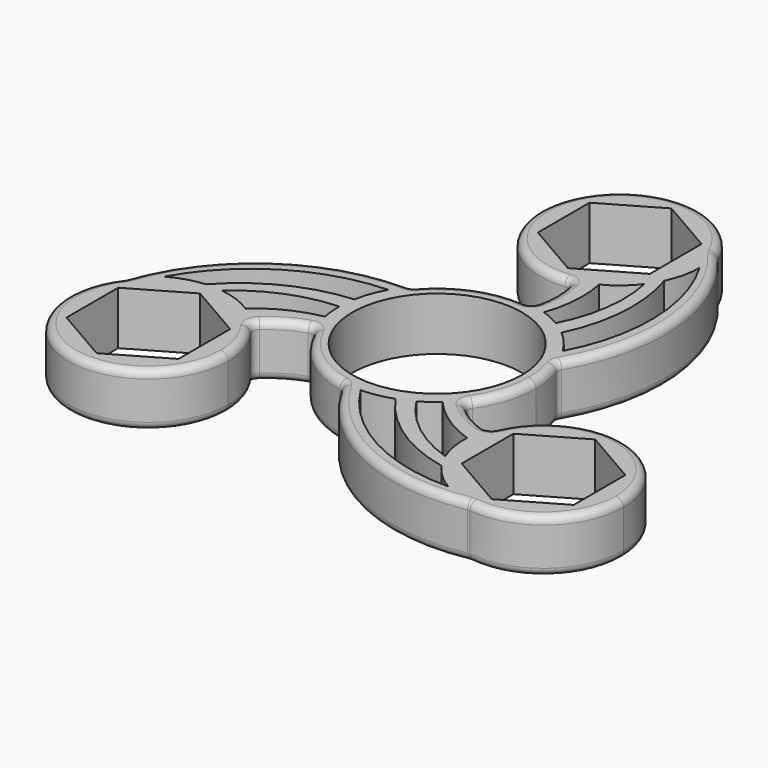
from build123d import *

# Parameters (mm, degrees)
F0_R     = 11.15
F1_DEPTH = 7
F2_R     = 1


with BuildPart() as f1:
    # F0 (on Top) → F1 (new body)
    with BuildSketch(Plane.XY):
        with BuildLine():
            ThreePointArc((-11.4217360903, 6.2083769767), (-10.7651051073, 7.2878331504), (-10.0067859301, 8.2984477674))
            ThreePointArc((-10.0067859301, 8.2984477674), (-24.8747570985, 3.8510516113), (-34.2433879176, -8.5208785455))
            ThreePointArc((-34.2433879176, -8.5208785455), (-32.8623464459, -7.069439044), (-31.2307621135, -5.9067332603))
            ThreePointArc((-31.2307621135, -5.9067332603), (-22.9201483535, 2.7569551195), (-11.4217360903, 6.2083769767))
        make_face()
        with BuildLine():
            ThreePointArc((-12.9988117388, 0.1757651253), (-12.936896451, 1.2793397577), (-12.7814596137, 2.3736659713))
            ThreePointArc((-12.7814596137, 2.3736659713), (-20.4515190805, 0.2762194234), (-26.7856148565, -4.5308924897))
            ThreePointArc((-26.7856148565, -4.5308924897), (-25.7070937202, -4.5035670054), (-24.6314618134, -4.5870566745))
            ThreePointArc((-24.6314618134, -4.5870566745), (-19.2285330831, -1.1959723533), (-12.9988117388, 0.1757651253))
        make_face()
        with BuildLine():
            ThreePointArc((-18.0539765779, -8.1140671604), (-15.3384929239, -5.9704194589), (-12.1242977306, -4.6905654818))
            ThreePointArc((-12.1242977306, -4.6905654818), (-12.4885737373, -3.6104744852), (-12.7568359951, -2.5026256999))
            ThreePointArc((-12.7568359951, -2.5026256999), (-16.7613572368, -3.8405452144), (-20.2703349988, -6.1885856886))
            ThreePointArc((-20.2703349988, -6.1885856886), (-19.0945249739, -7.0734788174), (-18.0539765779, -8.1140671604))
        make_face()
        with BuildLine():
            ThreePointArc((-31.2307621135, -5.9067332603), (-32.8623464459, -7.069439044), (-34.2433879176, -8.5208785455))
            ThreePointArc((-34.2433879176, -8.5208785455), (-29.4080372015, -24.9249073281), (-15.4807621135, -15))
            ThreePointArc((-15.4807621135, -15), (-16.1450809443, -11.3244897038), (-18.0539765779, -8.1140671604))
            ThreePointArc((-18.0539765779, -8.1140671604), (-19.0945249739, -7.0734788174), (-20.2703349988, -6.1885856886))
            ThreePointArc((-20.2703349988, -6.1885856886), (-22.3612094355, -5.143588969), (-24.6314618134, -4.5870566745))
            ThreePointArc((-24.6314618134, -4.5870566745), (-25.7070937202, -4.5035670054), (-26.7856148565, -4.5308924897))
            ThreePointArc((-26.7856148565, -4.5308924897), (-29.0853627145, -4.9694738369), (-31.2307621135, -5.9067332603))
        make_face()
        Polygon((-25.9807621135, -23.5), (-33.3419780457, -19.25), (-33.3419780457, -10.75), (-25.9807621135, -6.5), (-18.6195461814, -10.75), (-18.6195461814, -19.25), align=None, mode=Mode.SUBTRACT)
        with BuildLine():
            ThreePointArc((10.1242977306, -8.1546670969), (12.2600136725, -4.3234320569), (13, 0))
            ThreePointArc((13, 0), (12.7959129035, 2.2944744423), (12.1900595436, 4.516906942))
            ThreePointArc((12.1900595436, 4.516906942), (11.6940012005, 5.6789379222), (11.0874802232, 6.7873251211))
            ThreePointArc((11.0874802232, 6.7873251211), (9.8887607408, 8.4387446348), (8.4463848381, 9.8822357373))
            ThreePointArc((8.4463848381, 9.8822357373), (7.5763889557, 10.5640110939), (6.651622933, 11.1694186222))
            ThreePointArc((6.651622933, 11.1694186222), (5.460641215, 11.7975165828), (4.2110805653, 12.2990568936))
            ThreePointArc((4.2110805653, 12.2990568936), (3.1175242448, 12.6206593561), (2, 12.8452325787))
            ThreePointArc((2, 12.8452325787), (-4.6038536318, 12.1574887101), (-10.0067859301, 8.2984477674))
            ThreePointArc((-10.0067859301, 8.2984477674), (-10.7651051073, 7.2878331504), (-11.4217360903, 6.2083769767))
            ThreePointArc((-11.4217360903, 6.2083769767), (-12.2525476002, 4.3445456961), (-12.7814596137, 2.3736659713))
            ThreePointArc((-12.7814596137, 2.3736659713), (-12.936896451, 1.2793397577), (-12.9988117388, 0.1757651253))
            ThreePointArc((-12.9988117388, 0.1757651253), (-12.9472696698, -1.1697042782), (-12.7568359951, -2.5026256999))
            ThreePointArc((-12.7568359951, -2.5026256999), (-12.4885737373, -3.6104744852), (-12.1242977306, -4.6905654818))
            ThreePointArc((-12.1242977306, -4.6905654818), (-8.2267672533, -10.0657985555), (-2.1832736135, -12.8153547094))
            ThreePointArc((-2.1832736135, -12.8153547094), (-0.9288960931, -12.9667710726), (0.3342558671, -12.9957020978))
            ThreePointArc((0.3342558671, -12.9957020978), (2.3637868594, -12.7832903309), (4.3350747756, -12.2559017086))
            ThreePointArc((4.3350747756, -12.2559017086), (5.3605074953, -11.8433508516), (6.3471888058, -11.3451837474))
            ThreePointArc((6.3471888058, -11.3451837474), (7.4866284548, -10.6278123045), (8.5457554298, -9.7964311937))
            ThreePointArc((8.5457554298, -9.7964311937), (9.3710494925, -9.010184871), (10.1242977306, -8.1546670969))
        make_face()
        Circle(F0_R, mode=Mode.SUBTRACT)
        with BuildLine():
            ThreePointArc((-2.1832736135, -12.8153547094), (9.1022700226, -23.4676973659), (24.5009912418, -25.3952045755))
            ThreePointArc((24.5009912418, -25.3952045755), (22.5534870256, -24.9249073281), (20.7307621135, -24.0932667397))
            ThreePointArc((20.7307621135, -24.0932667397), (9.0724810061, -21.2279082924), (0.3342558671, -12.9957020978))
            ThreePointArc((0.3342558671, -12.9957020978), (-0.9288960931, -12.9667710726), (-2.1832736135, -12.8153547094))
        make_face()
        with BuildLine():
            ThreePointArc((16.2882385154, -19.0379433255), (10.6500089817, -16.0544119509), (6.3471888058, -11.3451837474))
            ThreePointArc((6.3471888058, -11.3451837474), (5.3605074953, -11.8433508516), (4.3350747756, -12.2559017086))
            ThreePointArc((4.3350747756, -12.2559017086), (9.9865465026, -17.8496447814), (17.3166754262, -20.9315766769))
            ThreePointArc((17.3166754262, -20.9315766769), (16.7537502944, -20.0112127164), (16.2882385154, -19.0379433255))
        make_face()
        with BuildLine():
            ThreePointArc((16.0539765779, -11.5781687755), (12.8397813846, -10.2983147984), (10.1242977306, -8.1546670969))
            ThreePointArc((10.1242977306, -8.1546670969), (9.3710494925, -9.010184871), (8.5457554298, -9.7964311937))
            ThreePointArc((8.5457554298, -9.7964311937), (11.7066883385, -12.5954885618), (15.4946399192, -14.4603322079))
            ThreePointArc((15.4946399192, -14.4603322079), (15.673074836, -12.9996042919), (16.0539765779, -11.5781687755))
        make_face()
        with BuildLine():
            ThreePointArc((36.4807621135, -15), (27.7155174097, -4.6442950958), (16.0539765779, -11.5781687755))
            ThreePointArc((16.0539765779, -11.5781687755), (15.673074836, -12.9996042919), (15.4946399192, -14.4603322079))
            ThreePointArc((15.4946399192, -14.4603322079), (15.6350834316, -16.793580946), (16.2882385154, -19.0379433255))
            ThreePointArc((16.2882385154, -19.0379433255), (16.7537502944, -20.0112127164), (17.3166754262, -20.9315766769))
            ThreePointArc((17.3166754262, -20.9315766769), (18.8463719434, -22.7039260706), (20.7307621135, -24.0932667397))
            ThreePointArc((20.7307621135, -24.0932667397), (22.5534870256, -24.9249073281), (24.5009912418, -25.3952045755))
            ThreePointArc((24.5009912418, -25.3952045755), (32.8623464459, -22.930560956), (36.4807621135, -15))
        make_face()
        Polygon((33.3419780457, -10.75), (33.3419780457, -19.25), (25.9807621135, -23.5), (18.6195461814, -19.25), (18.6195461814, -10.75), (25.9807621135, -6.5), align=None, mode=Mode.SUBTRACT)
        with BuildLine():
            ThreePointArc((11.0874802232, 6.7873251211), (11.6940012005, 5.6789379222), (12.1900595436, 4.516906942))
            ThreePointArc((12.1900595436, 4.516906942), (15.7724870759, 19.6166457546), (9.7423966758, 33.9160831211))
            ThreePointArc((9.7423966758, 33.9160831211), (10.3088594203, 31.9943463721), (10.5, 30))
            ThreePointArc((10.5, 30), (13.8476673473, 18.4709531729), (11.0874802232, 6.7873251211))
        make_face()
        with BuildLine():
            ThreePointArc((6.651622933, 11.1694186222), (7.5763889557, 10.5640110939), (8.4463848381, 9.8822357373))
            ThreePointArc((8.4463848381, 9.8822357373), (10.4649725779, 17.573425358), (9.4689394304, 25.4624691666))
            ThreePointArc((9.4689394304, 25.4624691666), (8.9533434258, 24.5147797218), (8.343223298, 23.625))
            ThreePointArc((8.343223298, 23.625), (8.5785241014, 17.2503843041), (6.651622933, 11.1694186222))
        make_face()
        with BuildLine():
            ThreePointArc((4.7756950796, 20.6489178965), (3.4214501379, 20.0730831094), (2, 19.692235936))
            ThreePointArc((2, 19.692235936), (2.4987115393, 16.2687342573), (2, 12.8452325787))
            ThreePointArc((2, 12.8452325787), (3.1175242448, 12.6206593561), (4.2110805653, 12.2990568936))
            ThreePointArc((4.2110805653, 12.2990568936), (5.0546688984, 16.4360337762), (4.7756950796, 20.6489178965))
        make_face()
        with BuildLine():
            ThreePointArc((10.5, 30), (10.3088594203, 31.9943463721), (9.7423966758, 33.9160831211))
            ThreePointArc((9.7423966758, 33.9160831211), (-9.2222788458, 35.0199176179), (2, 19.692235936))
            ThreePointArc((2, 19.692235936), (3.4214501379, 20.0730831094), (4.7756950796, 20.6489178965))
            ThreePointArc((4.7756950796, 20.6489178965), (6.726126004, 21.937169915), (8.343223298, 23.625))
            ThreePointArc((8.343223298, 23.625), (8.9533434258, 24.5147797218), (9.4689394304, 25.4624691666))
            ThreePointArc((9.4689394304, 25.4624691666), (10.238990771, 27.6733999075), (10.5, 30))
        make_face()
        Polygon((-7.3612159322, 34.25), (0, 38.5), (7.3612159322, 34.25), (7.3612159322, 25.75), (0, 21.5), (-7.3612159322, 25.75), align=None, mode=Mode.SUBTRACT)
    extrude(amount=F1_DEPTH)

    # F2
    f2_edges = [f1.edges().sort_by_distance(p)[0] for p in [
        (-34.243388, -8.520879, 3.5),
        (-18.053977, -8.114067, 3.5),
        (-25.716999, -25.496687, 0),
        (-25.716999, -25.496687, 7),
        (-12.124298, -4.690565, 3.5),
        (-2.183274, -12.815355, 3.5),
        (-8.226767, -10.065799, 0),
        (-8.226767, -10.065799, 7),
        (-15.338493, -5.970419, 0),
        (-15.338493, -5.970419, 7),
        (24.500991, -25.395205, 3.5),
        (9.10227, -23.467697, 0),
        (9.10227, -23.467697, 7),
        (16.053977, -11.578169, 3.5),
        (34.939278, -9.523231, 0),
        (34.939278, -9.523231, 7),
        (10.124298, -8.154667, 3.5),
        (12.839781, -10.298315, 0),
        (12.839781, -10.298315, 7),
        (12.19006, 4.516907, 3.5),
        (12.830621, -2.09169, 0),
        (12.830621, -2.09169, 7),
        (9.742397, 33.916083, 3.5),
        (15.772487, 19.616646, 0),
        (15.772487, 19.616646, 7),
        (2, 19.692236, 3.5),
        (-9.222279, 35.019918, 0),
        (-9.222279, 35.019918, 7),
        (2, 12.845233, 3.5),
        (2.498712, 16.268734, 0),
        (2.498712, 16.268734, 7),
        (-10.006786, 8.298448, 3.5),
        (-4.603854, 12.157489, 0),
        (-4.603854, 12.157489, 7),
        (-24.874757, 3.851052, 0),
        (-24.874757, 3.851052, 7),
    ]]
    fillet(f2_edges, radius=F2_R)


solid = f1.part
